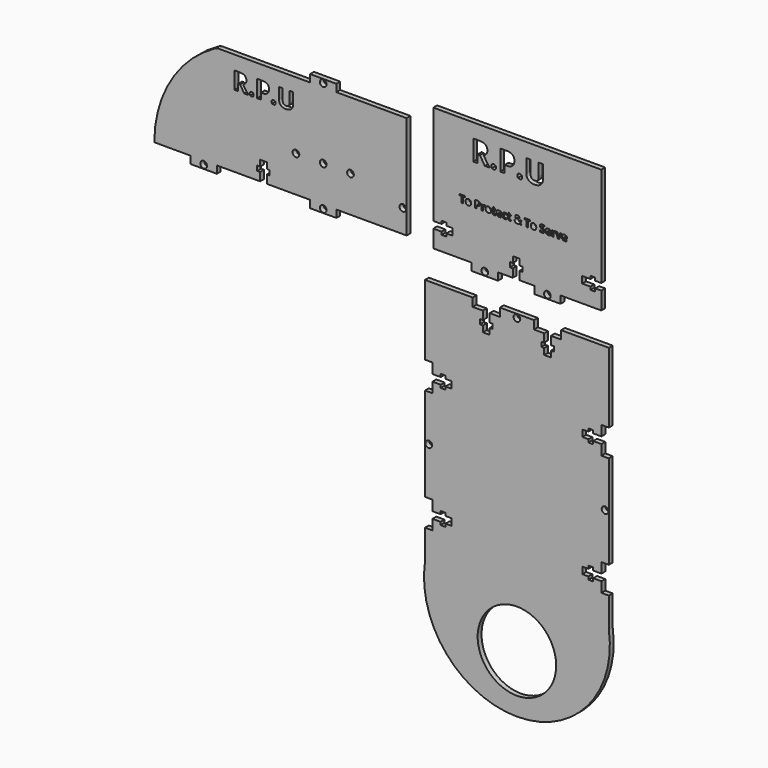
from build123d import *

# Parameters (mm, degrees)
F0_R     = 2.0574
F1_DEPTH = 2.9718
F2_R     = 2.0574
F3_DEPTH = 2.9718
F4_R     = 2.0574
F4_R_2   = 24.13
F5_DEPTH = 2.9718
F8_R     = 5.08


# Not quite as in the source:
# - ends of sketch curves that miss each other by under 0.0002 mm in the source are joined
# - a feature names something its author has since deleted; it is built from what else it names


with BuildPart() as f1:
    # F0 (on Front) → F1 (new body)
    with BuildSketch(Plane.XZ):
        Polygon((-18.5969026979, -10.7412008894), (-18.5969026979, -15.2876914638), (-2.4300471224, -15.2876914638), (-2.4300471224, -10.7412008894), (6.6548, -10.7412008894), (6.6548, -5.6612008894), (4.8768, -5.6612008894), (4.8768, -2.7392187621), (6.6548, -2.7392187621), (6.6548, 0.9935991106), (10.7696, 0.9935991106), (10.7696, -2.7392187621), (12.5476, -2.7392187621), (12.5476, -5.6612008894), (10.7696, -5.6612008894), (10.7696, -10.7412008894), (19.8544471224, -10.7412008894), (19.8544471224, -15.2876914638), (36.0213026979, -15.2876914638), (36.0213026979, -10.7412008894), (58.0559210762, -10.7412008894), (61.0555037856, -10.7412008894), (61.0555037856, -6.2738), (61.0555037856, 0), (57.3217037856, 0), (57.3217037856, -1.778), (54.4007037856, -1.778), (54.4007037856, 0), (49.3207037856, 0), (49.3207037856, 4.1148), (54.4007037856, 4.1148), (54.4007037856, 5.8928), (57.3051609099, 5.8928), (57.3051609099, 4.1148), (61.0555037856, 4.1148), (61.0555037856, 10.3886), (61.0555037856, 65.4587991106), (-42.2221365774, 65.4587991106), (-42.2221365774, 10.3886), (-42.2221365774, 4.1148), (-37.1421365774, 4.1148), (-37.1421365774, 5.8928905055), (-34.2144520407, 5.8928905055), (-34.2144520407, 4.1148), (-30.4746365774, 4.1148), (-30.4746365774, 0), (-34.2144520407, 0), (-34.2144520407, -1.7524508294), (-37.1421365774, -1.7524508294), (-37.1421365774, 0), (-42.2221365774, 0), (-42.2221365774, -6.2738), (-42.2221365774, -10.7412008894), (-38.2601322443, -10.7412008894), align=None)
        with Locations((-10.5134749102, -12.9762914638)):
            Circle(F0_R, mode=Mode.SUBTRACT)
        Polygon((-23.9621248782, 23.1793641805), (-23.9621248782, 19.4944459945), (-24.9110182404, 19.4944459945), (-24.9110182404, 23.1793641805), (-26.1262676342, 23.1793641805), (-26.1262676342, 23.9686397739), (-22.7478547345, 23.9686397739), (-22.7478547345, 23.1793641805), align=None, mode=Mode.SUBTRACT)
        with BuildLine():
            add(Edge.make_bspline(
                [(-19.2254920678, 22.1506619338), (-19.0237665439, 21.7496590113), (-19.0237665439, 21.2110714476)],
                knots=[0, 0, 0, 1, 1, 1], degree=2))
            add(Edge.make_bspline(
                [(-19.0237665439, 21.2110714476), (-19.0237665439, 20.3757710988), (-19.464429096, 19.904262168)],
                knots=[0, 0, 0, 1, 1, 1], degree=2))
            add(Edge.make_bspline(
                [(-19.464429096, 19.904262168), (-19.9050916482, 19.4327532372), (-20.6914294912, 19.4327532372)],
                knots=[0, 0, 0, 1, 1, 1], degree=2))
            add(Edge.make_bspline(
                [(-20.6914294912, 19.4327532372), (-21.1839922995, 19.4327532372), (-21.560513969, 19.6486778877)],
                knots=[0, 0, 0, 1, 1, 1], degree=2))
            add(Edge.make_bspline(
                [(-21.560513969, 19.6486778877), (-21.9370356386, 19.8646025383), (-22.1387611624, 20.2685432111)],
                knots=[0, 0, 0, 1, 1, 1], degree=2))
            add(Edge.make_bspline(
                [(-22.1387611624, 20.2685432111), (-22.3404866863, 20.6724838839), (-22.3404866863, 21.2110714476)],
                knots=[0, 0, 0, 1, 1, 1], degree=2))
            add(Edge.make_bspline(
                [(-22.3404866863, 21.2110714476), (-22.3404866863, 22.0493095468), (-21.9032515096, 22.5144533518)],
                knots=[0, 0, 0, 1, 1, 1], degree=2))
            add(Edge.make_bspline(
                [(-21.9032515096, 22.5144533518), (-21.4660163329, 22.9795971568), (-20.672823739, 22.9795971568)],
                knots=[0, 0, 0, 1, 1, 1], degree=2))
            add(Edge.make_bspline(
                [(-20.672823739, 22.9795971568), (-20.1802609307, 22.9795971568), (-19.8037392612, 22.7656310065)],
                knots=[0, 0, 0, 1, 1, 1], degree=2))
            add(Edge.make_bspline(
                [(-19.8037392612, 22.7656310065), (-19.4272175916, 22.5516648562), (-19.2254920678, 22.1506619338)],
                knots=[0, 0, 0, 1, 1, 1], degree=2))
        make_face(mode=Mode.SUBTRACT)
        with BuildLine():
            add(Edge.make_bspline(
                [(-13.8831930607, 23.6180682324), (-13.4596673856, 23.2674966909), (-13.4596673856, 22.5732083588)],
                knots=[0, 0, 0, 1, 1, 1], degree=2))
            add(Edge.make_bspline(
                [(-13.4596673856, 22.5732083588), (-13.4596673856, 21.8505217733), (-13.911101689, 21.468124603)],
                knots=[0, 0, 0, 1, 1, 1], degree=2))
            add(Edge.make_bspline(
                [(-13.911101689, 21.468124603), (-14.3625359924, 21.0857274328), (-15.1948985909, 21.0857274328)],
                knots=[0, 0, 0, 1, 1, 1], degree=2))
            Line((-15.1948985909, 21.0857274328), (-15.601287389, 21.0857274328))
            Line((-15.601287389, 21.0857274328), (-15.601287389, 19.4944459945))
            Line((-15.601287389, 19.4944459945), (-16.5501807512, 19.4944459945))
            Line((-16.5501807512, 19.4944459945), (-16.5501807512, 23.9686397739))
            Line((-16.5501807512, 23.9686397739), (-15.1214548322, 23.9686397739))
            add(Edge.make_bspline(
                [(-15.1214548322, 23.9686397739), (-14.3067187358, 23.9686397739), (-13.8831930607, 23.6180682324)],
                knots=[0, 0, 0, 1, 1, 1], degree=2))
        make_face(mode=Mode.SUBTRACT)
        with BuildLine():
            add(Edge.make_bspline(
                [(-11.367499513, 22.803821761), (-11.096736856, 22.9795971568), (-10.7784805684, 22.9795971568)],
                knots=[0, 0, 0, 1, 1, 1], degree=2))
            add(Edge.make_bspline(
                [(-10.7784805684, 22.9795971568), (-10.5885060459, 22.9795971568), (-10.4631620311, 22.9521781536)],
                knots=[0, 0, 0, 1, 1, 1], degree=2))
            Line((-10.4631620311, 22.9521781536), (-10.5336680394, 22.0777078001))
            add(Edge.make_bspline(
                [(-10.5336680394, 22.0777078001), (-10.6472610528, 22.1080645537), (-10.8088373219, 22.1080645537)],
                knots=[0, 0, 0, 1, 1, 1], degree=2))
            add(Edge.make_bspline(
                [(-10.8088373219, 22.1080645537), (-11.2553753748, 22.1080645537), (-11.5050841543, 21.8784304016)],
                knots=[0, 0, 0, 1, 1, 1], degree=2))
            add(Edge.make_bspline(
                [(-11.5050841543, 21.8784304016), (-11.7547929339, 21.6487962494), (-11.7547929339, 21.2355527005)],
                knots=[0, 0, 0, 1, 1, 1], degree=2))
            Line((-11.7547929339, 21.2355527005), (-11.7547929339, 19.4944459945))
            Line((-11.7547929339, 19.4944459945), (-12.6880182943, 19.4944459945))
            Line((-12.6880182943, 19.4944459945), (-12.6880182943, 22.9159458993))
            Line((-12.6880182943, 22.9159458993), (-11.9809997106, 22.9159458993))
            Line((-11.9809997106, 22.9159458993), (-11.8429254443, 22.3401468312))
            Line((-11.8429254443, 22.3401468312), (-11.797879939, 22.3401468312))
            add(Edge.make_bspline(
                [(-11.797879939, 22.3401468312), (-11.6382621701, 22.6280463652), (-11.367499513, 22.803821761)],
                knots=[0, 0, 0, 1, 1, 1], degree=2))
        make_face(mode=Mode.SUBTRACT)
        with BuildLine():
            add(Edge.make_bspline(
                [(-6.9349238636, 22.1506619338), (-6.7331983397, 21.7496590113), (-6.7331983397, 21.2110714476)],
                knots=[0, 0, 0, 1, 1, 1], degree=2))
            add(Edge.make_bspline(
                [(-6.7331983397, 21.2110714476), (-6.7331983397, 20.3757710988), (-7.1738608919, 19.904262168)],
                knots=[0, 0, 0, 1, 1, 1], degree=2))
            add(Edge.make_bspline(
                [(-7.1738608919, 19.904262168), (-7.614523444, 19.4327532372), (-8.400861287, 19.4327532372)],
                knots=[0, 0, 0, 1, 1, 1], degree=2))
            add(Edge.make_bspline(
                [(-8.400861287, 19.4327532372), (-8.8934240953, 19.4327532372), (-9.2699457649, 19.6486778877)],
                knots=[0, 0, 0, 1, 1, 1], degree=2))
            add(Edge.make_bspline(
                [(-9.2699457649, 19.6486778877), (-9.6464674344, 19.8646025383), (-9.8481929583, 20.2685432111)],
                knots=[0, 0, 0, 1, 1, 1], degree=2))
            add(Edge.make_bspline(
                [(-9.8481929583, 20.2685432111), (-10.0499184822, 20.6724838839), (-10.0499184822, 21.2110714476)],
                knots=[0, 0, 0, 1, 1, 1], degree=2))
            add(Edge.make_bspline(
                [(-10.0499184822, 21.2110714476), (-10.0499184822, 22.0493095468), (-9.6126833054, 22.5144533518)],
                knots=[0, 0, 0, 1, 1, 1], degree=2))
            add(Edge.make_bspline(
                [(-9.6126833054, 22.5144533518), (-9.1754481287, 22.9795971568), (-8.3822555348, 22.9795971568)],
                knots=[0, 0, 0, 1, 1, 1], degree=2))
            add(Edge.make_bspline(
                [(-8.3822555348, 22.9795971568), (-7.8896927266, 22.9795971568), (-7.513171057, 22.7656310065)],
                knots=[0, 0, 0, 1, 1, 1], degree=2))
            add(Edge.make_bspline(
                [(-7.513171057, 22.7656310065), (-7.1366493875, 22.5516648562), (-6.9349238636, 22.1506619338)],
                knots=[0, 0, 0, 1, 1, 1], degree=2))
        make_face(mode=Mode.SUBTRACT)
        with BuildLine():
            add(Edge.make_bspline(
                [(-4.8158266129, 20.2719705865), (-4.7041920997, 20.1769833253), (-4.5200930779, 20.1769833253)],
                knots=[0, 0, 0, 1, 1, 1], degree=2))
            add(Edge.make_bspline(
                [(-4.5200930779, 20.1769833253), (-4.2752805489, 20.1769833253), (-3.9325430084, 20.2837215879)],
                knots=[0, 0, 0, 1, 1, 1], degree=2))
            Line((-3.9325430084, 20.2837215879), (-3.9325430084, 19.5894332557))
            add(Edge.make_bspline(
                [(-3.9325430084, 19.5894332557), (-4.2811560496, 19.4327532372), (-4.7893868598, 19.4327532372)],
                knots=[0, 0, 0, 1, 1, 1], degree=2))
            add(Edge.make_bspline(
                [(-4.7893868598, 19.4327532372), (-5.349517926, 19.4327532372), (-5.6051022063, 19.7162461457)],
                knots=[0, 0, 0, 1, 1, 1], degree=2))
            add(Edge.make_bspline(
                [(-5.6051022063, 19.7162461457), (-5.8606864865, 19.9997390543), (-5.8606864865, 20.5657456212)],
                knots=[0, 0, 0, 1, 1, 1], degree=2))
            Line((-5.8606864865, 20.5657456212), (-5.8606864865, 22.2148028164))
            Line((-5.8606864865, 22.2148028164), (-6.3072245393, 22.2148028164))
            Line((-6.3072245393, 22.2148028164), (-6.3072245393, 22.609440613))
            Line((-6.3072245393, 22.609440613), (-5.7931182285, 22.9218214))
            Line((-5.7931182285, 22.9218214), (-5.5238244467, 23.6445079855))
            Line((-5.5238244467, 23.6445079855), (-4.9274611261, 23.6445079855))
            Line((-4.9274611261, 23.6445079855), (-4.9274611261, 22.9159458993))
            Line((-4.9274611261, 22.9159458993), (-3.9697545128, 22.9159458993))
            Line((-3.9697545128, 22.9159458993), (-3.9697545128, 22.2148028164))
            Line((-3.9697545128, 22.2148028164), (-4.9274611261, 22.2148028164))
            Line((-4.9274611261, 22.2148028164), (-4.9274611261, 20.5657456212))
            add(Edge.make_bspline(
                [(-4.9274611261, 20.5657456212), (-4.9274611261, 20.3669578477), (-4.8158266129, 20.2719705865)],
                knots=[0, 0, 0, 1, 1, 1], degree=2))
        make_face(mode=Mode.SUBTRACT)
        with BuildLine():
            add(Edge.make_bspline(
                [(-1.013398413, 19.4924874943), (-1.2915054459, 19.4327532372), (-1.6929979934, 19.4327532372)],
                knots=[0, 0, 0, 1, 1, 1], degree=2))
            add(Edge.make_bspline(
                [(-1.6929979934, 19.4327532372), (-2.5185058411, 19.4327532372), (-2.9836496461, 19.8890837912)],
                knots=[0, 0, 0, 1, 1, 1], degree=2))
            add(Edge.make_bspline(
                [(-2.9836496461, 19.8890837912), (-3.4487934511, 20.3454143452), (-3.4487934511, 21.180714694)],
                knots=[0, 0, 0, 1, 1, 1], degree=2))
            add(Edge.make_bspline(
                [(-3.4487934511, 21.180714694), (-3.4487934511, 22.0404962957), (-3.0189026503, 22.5100467263)],
                knots=[0, 0, 0, 1, 1, 1], degree=2))
            add(Edge.make_bspline(
                [(-3.0189026503, 22.5100467263), (-2.5890118494, 22.9795971568), (-1.8300930096, 22.9795971568)],
                knots=[0, 0, 0, 1, 1, 1], degree=2))
            add(Edge.make_bspline(
                [(-1.8300930096, 22.9795971568), (-1.1054479239, 22.9795971568), (-0.7015072511, 22.566843233)],
                knots=[0, 0, 0, 1, 1, 1], degree=2))
            add(Edge.make_bspline(
                [(-0.7015072511, 22.566843233), (-0.2975665783, 22.1540893092), (-0.2975665783, 21.425527223)],
                knots=[0, 0, 0, 1, 1, 1], degree=2))
            Line((-0.2975665783, 21.425527223), (-0.2975665783, 20.9721344193))
            Line((-0.2975665783, 20.9721344193), (-2.5038170893, 20.9721344193))
            add(Edge.make_bspline(
                [(-2.5038170893, 20.9721344193), (-2.4881490875, 20.5745588723), (-2.2678178114, 20.3512898459)],
                knots=[0, 0, 0, 1, 1, 1], degree=2))
            add(Edge.make_bspline(
                [(-2.2678178114, 20.3512898459), (-2.0474865354, 20.1280208195), (-1.6499109883, 20.1280208195)],
                knots=[0, 0, 0, 1, 1, 1], degree=2))
            add(Edge.make_bspline(
                [(-1.6499109883, 20.1280208195), (-1.3404679517, 20.1280208195), (-1.0652986691, 20.192161702)],
                knots=[0, 0, 0, 1, 1, 1], degree=2))
            add(Edge.make_bspline(
                [(-1.0652986691, 20.192161702), (-0.7901293866, 20.2563025846), (-0.4904788511, 20.3973146013)],
                knots=[0, 0, 0, 1, 1, 1], degree=2))
            Line((-0.4904788511, 20.3973146013), (-0.4904788511, 19.6746280158))
            add(Edge.make_bspline(
                [(-0.4904788511, 19.6746280158), (-0.7352913801, 19.5522217513), (-1.013398413, 19.4924874943)],
                knots=[0, 0, 0, 1, 1, 1], degree=2))
        make_face(mode=Mode.SUBTRACT)
        with BuildLine():
            add(Edge.make_bspline(
                [(2.4335619948, 19.4880808687), (2.2024589675, 19.4327532372), (1.8509081759, 19.4327532372)],
                knots=[0, 0, 0, 1, 1, 1], degree=2))
            add(Edge.make_bspline(
                [(1.8509081759, 19.4327532372), (0.2537512369, 19.4327532372), (0.2537512369, 21.1865901947)],
                knots=[0, 0, 0, 1, 1, 1], degree=2))
            add(Edge.make_bspline(
                [(0.2537512369, 21.1865901947), (0.2537512369, 22.0591020479), (0.6880486633, 22.5193496024)],
                knots=[0, 0, 0, 1, 1, 1], degree=2))
            add(Edge.make_bspline(
                [(0.6880486633, 22.5193496024), (1.1223460897, 22.9795971568), (1.9331651856, 22.9795971568)],
                knots=[0, 0, 0, 1, 1, 1], degree=2))
            add(Edge.make_bspline(
                [(1.9331651856, 22.9795971568), (2.5265907558, 22.9795971568), (2.9985893117, 22.7475148794)],
                knots=[0, 0, 0, 1, 1, 1], degree=2))
            Line((2.9985893117, 22.7475148794), (2.722440779, 22.0248282939))
            add(Edge.make_bspline(
                [(2.722440779, 22.0248282939), (2.5021095029, 22.1139400544), (2.3126246055, 22.1707365611)],
                knots=[0, 0, 0, 1, 1, 1], degree=2))
            add(Edge.make_bspline(
                [(2.3126246055, 22.1707365611), (2.1231397081, 22.2275330679), (1.9331651856, 22.2275330679)],
                knots=[0, 0, 0, 1, 1, 1], degree=2))
            add(Edge.make_bspline(
                [(1.9331651856, 22.2275330679), (1.2046030994, 22.2275330679), (1.2046030994, 21.1924656954)],
                knots=[0, 0, 0, 1, 1, 1], degree=2))
            add(Edge.make_bspline(
                [(1.2046030994, 21.1924656954), (1.2046030994, 20.1887343266), (1.9331651856, 20.1887343266)],
                knots=[0, 0, 0, 1, 1, 1], degree=2))
            add(Edge.make_bspline(
                [(1.9331651856, 20.1887343266), (2.2024589675, 20.1887343266), (2.4320931196, 20.2607092102)],
                knots=[0, 0, 0, 1, 1, 1], degree=2))
            add(Edge.make_bspline(
                [(2.4320931196, 20.2607092102), (2.6617272718, 20.3326840937), (2.8908717989, 20.4864263619)],
                knots=[0, 0, 0, 1, 1, 1], degree=2))
            Line((2.8908717989, 20.4864263619), (2.8908717989, 19.6873582673))
            add(Edge.make_bspline(
                [(2.8908717989, 19.6873582673), (2.6646650222, 19.5434085003), (2.4335619948, 19.4880808687)],
                knots=[0, 0, 0, 1, 1, 1], degree=2))
        make_face(mode=Mode.SUBTRACT)
        with BuildLine():
            add(Edge.make_bspline(
                [(4.8297870283, 20.2719705865), (4.9414215415, 20.1769833253), (5.1255205633, 20.1769833253)],
                knots=[0, 0, 0, 1, 1, 1], degree=2))
            add(Edge.make_bspline(
                [(5.1255205633, 20.1769833253), (5.3703330923, 20.1769833253), (5.7130706328, 20.2837215879)],
                knots=[0, 0, 0, 1, 1, 1], degree=2))
            Line((5.7130706328, 20.2837215879), (5.7130706328, 19.5894332557))
            add(Edge.make_bspline(
                [(5.7130706328, 19.5894332557), (5.3644575916, 19.4327532372), (4.8562267815, 19.4327532372)],
                knots=[0, 0, 0, 1, 1, 1], degree=2))
            add(Edge.make_bspline(
                [(4.8562267815, 19.4327532372), (4.2960957152, 19.4327532372), (4.0405114349, 19.7162461457)],
                knots=[0, 0, 0, 1, 1, 1], degree=2))
            add(Edge.make_bspline(
                [(4.0405114349, 19.7162461457), (3.7849271547, 19.9997390543), (3.7849271547, 20.5657456212)],
                knots=[0, 0, 0, 1, 1, 1], degree=2))
            Line((3.7849271547, 20.5657456212), (3.7849271547, 22.2148028164))
            Line((3.7849271547, 22.2148028164), (3.3383891019, 22.2148028164))
            Line((3.3383891019, 22.2148028164), (3.3383891019, 22.609440613))
            Line((3.3383891019, 22.609440613), (3.8524954127, 22.9218214))
            Line((3.8524954127, 22.9218214), (4.1217891946, 23.6445079855))
            Line((4.1217891946, 23.6445079855), (4.7181525151, 23.6445079855))
            Line((4.7181525151, 23.6445079855), (4.7181525151, 22.9159458993))
            Line((4.7181525151, 22.9159458993), (5.6758591284, 22.9159458993))
            Line((5.6758591284, 22.9159458993), (5.6758591284, 22.2148028164))
            Line((5.6758591284, 22.2148028164), (4.7181525151, 22.2148028164))
            Line((4.7181525151, 22.2148028164), (4.7181525151, 20.5657456212))
            add(Edge.make_bspline(
                [(4.7181525151, 20.5657456212), (4.7181525151, 20.3669578477), (4.8297870283, 20.2719705865)],
                knots=[0, 0, 0, 1, 1, 1], degree=2))
        make_face(mode=Mode.SUBTRACT)
        with Locations((27.9378749102, -12.9762914638)):
            Circle(F0_R, mode=Mode.SUBTRACT)
        with BuildLine():
            Line((11.3222152965, 20.3914391006), (12.2436896555, 19.4944459945))
            Line((12.2436896555, 19.4944459945), (11.090133019, 19.4944459945))
            Line((11.090133019, 19.4944459945), (10.7385822274, 19.8401212854))
            add(Edge.make_bspline(
                [(10.7385822274, 19.8401212854), (10.1539699083, 19.4327532372), (9.416594571, 19.4327532372)],
                knots=[0, 0, 0, 1, 1, 1], degree=2))
            add(Edge.make_bspline(
                [(9.416594571, 19.4327532372), (8.6694267326, 19.4327532372), (8.2317019308, 19.7759804028)],
                knots=[0, 0, 0, 1, 1, 1], degree=2))
            add(Edge.make_bspline(
                [(8.2317019308, 19.7759804028), (7.793977129, 20.1192075684), (7.793977129, 20.7028406375)],
                knots=[0, 0, 0, 1, 1, 1], degree=2))
            add(Edge.make_bspline(
                [(7.793977129, 20.7028406375), (7.793977129, 21.1229389372), (7.9790554009, 21.4181828471)],
                knots=[0, 0, 0, 1, 1, 1], degree=2))
            add(Edge.make_bspline(
                [(7.9790554009, 21.4181828471), (8.1641336728, 21.713426757), (8.6145887261, 21.9699902874)],
                knots=[0, 0, 0, 1, 1, 1], degree=2))
            add(Edge.make_bspline(
                [(8.6145887261, 21.9699902874), (8.3844649489, 22.2334085686), (8.2806644366, 22.473814472)],
                knots=[0, 0, 0, 1, 1, 1], degree=2))
            add(Edge.make_bspline(
                [(8.2806644366, 22.473814472), (8.1768639243, 22.7142203754), (8.1768639243, 22.998202909)],
                knots=[0, 0, 0, 1, 1, 1], degree=2))
            add(Edge.make_bspline(
                [(8.1768639243, 22.998202909), (8.1768639243, 23.4633467141), (8.5333109665, 23.7478188727)],
                knots=[0, 0, 0, 1, 1, 1], degree=2))
            add(Edge.make_bspline(
                [(8.5333109665, 23.7478188727), (8.8897580087, 24.0322910314), (9.4861213292, 24.0322910314)],
                knots=[0, 0, 0, 1, 1, 1], degree=2))
            add(Edge.make_bspline(
                [(9.4861213292, 24.0322910314), (10.0560448967, 24.0322910314), (10.3973135621, 23.7678935001)],
                knots=[0, 0, 0, 1, 1, 1], degree=2))
            add(Edge.make_bspline(
                [(10.3973135621, 23.7678935001), (10.7385822274, 23.5034959688), (10.7385822274, 23.0598956663)],
                knots=[0, 0, 0, 1, 1, 1], degree=2))
            add(Edge.make_bspline(
                [(10.7385822274, 23.0598956663), (10.7385822274, 22.6956146232), (10.5270642024, 22.3940055876)],
                knots=[0, 0, 0, 1, 1, 1], degree=2))
            add(Edge.make_bspline(
                [(10.5270642024, 22.3940055876), (10.3155461774, 22.0923965519), (9.8445268717, 21.8201650197)],
                knots=[0, 0, 0, 1, 1, 1], degree=2))
            Line((9.8445268717, 21.8201650197), (10.7141009745, 20.9721344193))
            add(Edge.make_bspline(
                [(10.7141009745, 20.9721344193), (10.9305152501, 21.3305399617), (11.090133019, 21.8936087784)],
                knots=[0, 0, 0, 1, 1, 1], degree=2))
            Line((11.090133019, 21.8936087784), (12.0635076342, 21.8936087784))
            add(Edge.make_bspline(
                [(12.0635076342, 21.8936087784), (11.9528523711, 21.4803652295), (11.7599400983, 21.0871963079)],
                knots=[0, 0, 0, 1, 1, 1], degree=2))
            add(Edge.make_bspline(
                [(11.7599400983, 21.0871963079), (11.5670278254, 20.6940273864), (11.3222152965, 20.3914391006)],
                knots=[0, 0, 0, 1, 1, 1], degree=2))
        make_face(mode=Mode.SUBTRACT)
        Polygon((16.1616693691, 23.1793641805), (16.1616693691, 19.4944459945), (15.2127760068, 19.4944459945), (15.2127760068, 23.1793641805), (13.997526613, 23.1793641805), (13.997526613, 23.9686397739), (17.3759395127, 23.9686397739), (17.3759395127, 23.1793641805), align=None, mode=Mode.SUBTRACT)
        with BuildLine():
            add(Edge.make_bspline(
                [(20.8983021795, 22.1506619338), (21.1000277033, 21.7496590113), (21.1000277033, 21.2110714476)],
                knots=[0, 0, 0, 1, 1, 1], degree=2))
            add(Edge.make_bspline(
                [(21.1000277033, 21.2110714476), (21.1000277033, 20.3757710988), (20.6593651512, 19.904262168)],
                knots=[0, 0, 0, 1, 1, 1], degree=2))
            add(Edge.make_bspline(
                [(20.6593651512, 19.904262168), (20.2187025991, 19.4327532372), (19.432364756, 19.4327532372)],
                knots=[0, 0, 0, 1, 1, 1], degree=2))
            add(Edge.make_bspline(
                [(19.432364756, 19.4327532372), (18.9398019478, 19.4327532372), (18.5632802782, 19.6486778877)],
                knots=[0, 0, 0, 1, 1, 1], degree=2))
            add(Edge.make_bspline(
                [(18.5632802782, 19.6486778877), (18.1867586087, 19.8646025383), (17.9850330848, 20.2685432111)],
                knots=[0, 0, 0, 1, 1, 1], degree=2))
            add(Edge.make_bspline(
                [(17.9850330848, 20.2685432111), (17.7833075609, 20.6724838839), (17.7833075609, 21.2110714476)],
                knots=[0, 0, 0, 1, 1, 1], degree=2))
            add(Edge.make_bspline(
                [(17.7833075609, 21.2110714476), (17.7833075609, 22.0493095468), (18.2205427377, 22.5144533518)],
                knots=[0, 0, 0, 1, 1, 1], degree=2))
            add(Edge.make_bspline(
                [(18.2205427377, 22.5144533518), (18.6577779144, 22.9795971568), (19.4509705082, 22.9795971568)],
                knots=[0, 0, 0, 1, 1, 1], degree=2))
            add(Edge.make_bspline(
                [(19.4509705082, 22.9795971568), (19.9435333165, 22.9795971568), (20.3200549861, 22.7656310065)],
                knots=[0, 0, 0, 1, 1, 1], degree=2))
            add(Edge.make_bspline(
                [(20.3200549861, 22.7656310065), (20.6965766556, 22.5516648562), (20.8983021795, 22.1506619338)],
                knots=[0, 0, 0, 1, 1, 1], degree=2))
        make_face(mode=Mode.SUBTRACT)
        with BuildLine():
            add(Edge.make_bspline(
                [(25.982079156, 21.4759586039), (26.2146510585, 21.1748391933), (26.2146510585, 20.7371143915)],
                knots=[0, 0, 0, 1, 1, 1], degree=2))
            add(Edge.make_bspline(
                [(26.2146510585, 20.7371143915), (26.2146510585, 20.1309585698), (25.7783951319, 19.7818559035)],
                knots=[0, 0, 0, 1, 1, 1], degree=2))
            add(Edge.make_bspline(
                [(25.7783951319, 19.7818559035), (25.3421392052, 19.4327532372), (24.5655938634, 19.4327532372)],
                knots=[0, 0, 0, 1, 1, 1], degree=2))
            add(Edge.make_bspline(
                [(24.5655938634, 19.4327532372), (23.8487827786, 19.4327532372), (23.2984442134, 19.7030262692)],
                knots=[0, 0, 0, 1, 1, 1], degree=2))
            Line((23.2984442134, 19.7030262692), (23.2984442134, 20.5843513734))
            add(Edge.make_bspline(
                [(23.2984442134, 20.5843513734), (23.750857767, 20.3816465995), (24.0647074291, 20.2993895897)],
                knots=[0, 0, 0, 1, 1, 1], degree=2))
            add(Edge.make_bspline(
                [(24.0647074291, 20.2993895897), (24.3785570912, 20.21713258), (24.6390376221, 20.21713258)],
                knots=[0, 0, 0, 1, 1, 1], degree=2))
            add(Edge.make_bspline(
                [(24.6390376221, 20.21713258), (24.9504391589, 20.21713258), (25.1174013037, 20.3361114691)],
                knots=[0, 0, 0, 1, 1, 1], degree=2))
            add(Edge.make_bspline(
                [(25.1174013037, 20.3361114691), (25.2843634484, 20.4550903582), (25.2843634484, 20.6910896361)],
                knots=[0, 0, 0, 1, 1, 1], degree=2))
            add(Edge.make_bspline(
                [(25.2843634484, 20.6910896361), (25.2843634484, 20.8223091516), (25.2109196897, 20.9251304138)],
                knots=[0, 0, 0, 1, 1, 1], degree=2))
            add(Edge.make_bspline(
                [(25.2109196897, 20.9251304138), (25.137475931, 21.0279516759), (24.9949950392, 21.1224493121)],
                knots=[0, 0, 0, 1, 1, 1], degree=2))
            add(Edge.make_bspline(
                [(24.9949950392, 21.1224493121), (24.8525141473, 21.2169469483), (24.4147893455, 21.425527223)],
                knots=[0, 0, 0, 1, 1, 1], degree=2))
            add(Edge.make_bspline(
                [(24.4147893455, 21.425527223), (24.0054627971, 21.6184394958), (23.8003098978, 21.7956837668)],
                knots=[0, 0, 0, 1, 1, 1], degree=2))
            add(Edge.make_bspline(
                [(23.8003098978, 21.7956837668), (23.5951569986, 21.9729280377), (23.4727507341, 22.2089273157)],
                knots=[0, 0, 0, 1, 1, 1], degree=2))
            add(Edge.make_bspline(
                [(23.4727507341, 22.2089273157), (23.3503444696, 22.4449265936), (23.3503444696, 22.7592658808)],
                knots=[0, 0, 0, 1, 1, 1], degree=2))
            add(Edge.make_bspline(
                [(23.3503444696, 22.7592658808), (23.3503444696, 23.3536707011), (23.7528162672, 23.6929808662)],
                knots=[0, 0, 0, 1, 1, 1], degree=2))
            add(Edge.make_bspline(
                [(23.7528162672, 23.6929808662), (24.1552880648, 24.0322910314), (24.8652443988, 24.0322910314)],
                knots=[0, 0, 0, 1, 1, 1], degree=2))
            add(Edge.make_bspline(
                [(24.8652443988, 24.0322910314), (25.2138574401, 24.0322910314), (25.5306448526, 23.9500340217)],
                knots=[0, 0, 0, 1, 1, 1], degree=2))
            add(Edge.make_bspline(
                [(25.5306448526, 23.9500340217), (25.847432265, 23.8677770119), (26.1931075559, 23.7179517442)],
                knots=[0, 0, 0, 1, 1, 1], degree=2))
            Line((26.1931075559, 23.7179517442), (25.8875815198, 22.9795971568))
            add(Edge.make_bspline(
                [(25.8875815198, 22.9795971568), (25.5291759774, 23.1264846742), (25.2951351997, 23.1847500561)],
                knots=[0, 0, 0, 1, 1, 1], degree=2))
            add(Edge.make_bspline(
                [(25.2951351997, 23.1847500561), (25.061094422, 23.243015438), (24.8348876452, 23.243015438)],
                knots=[0, 0, 0, 1, 1, 1], degree=2))
            add(Edge.make_bspline(
                [(24.8348876452, 23.243015438), (24.5655938634, 23.243015438), (24.4216440963, 23.1176714232)],
                knots=[0, 0, 0, 1, 1, 1], degree=2))
            add(Edge.make_bspline(
                [(24.4216440963, 23.1176714232), (24.2776943293, 22.9923274083), (24.2776943293, 22.7906018845)],
                knots=[0, 0, 0, 1, 1, 1], degree=2))
            add(Edge.make_bspline(
                [(24.2776943293, 22.7906018845), (24.2776943293, 22.6652578697), (24.3359597112, 22.5717394836)],
                knots=[0, 0, 0, 1, 1, 1], degree=2))
            add(Edge.make_bspline(
                [(24.3359597112, 22.5717394836), (24.3942250931, 22.4782210975), (24.5210379831, 22.3910678372)],
                knots=[0, 0, 0, 1, 1, 1], degree=2))
            add(Edge.make_bspline(
                [(24.5210379831, 22.3910678372), (24.6478508731, 22.3039145769), (25.1218079292, 22.0777078001)],
                knots=[0, 0, 0, 1, 1, 1], degree=2))
            add(Edge.make_bspline(
                [(25.1218079292, 22.0777078001), (25.7495072534, 21.7770780146), (25.982079156, 21.4759586039)],
                knots=[0, 0, 0, 1, 1, 1], degree=2))
        make_face(mode=Mode.SUBTRACT)
        with BuildLine():
            add(Edge.make_bspline(
                [(29.1798204093, 19.4924874943), (28.9017133764, 19.4327532372), (28.5002208289, 19.4327532372)],
                knots=[0, 0, 0, 1, 1, 1], degree=2))
            add(Edge.make_bspline(
                [(28.5002208289, 19.4327532372), (27.6747129812, 19.4327532372), (27.2095691762, 19.8890837912)],
                knots=[0, 0, 0, 1, 1, 1], degree=2))
            add(Edge.make_bspline(
                [(27.2095691762, 19.8890837912), (26.7444253712, 20.3454143452), (26.7444253712, 21.180714694)],
                knots=[0, 0, 0, 1, 1, 1], degree=2))
            add(Edge.make_bspline(
                [(26.7444253712, 21.180714694), (26.7444253712, 22.0404962957), (27.174316172, 22.5100467263)],
                knots=[0, 0, 0, 1, 1, 1], degree=2))
            add(Edge.make_bspline(
                [(27.174316172, 22.5100467263), (27.6042069729, 22.9795971568), (28.3631258127, 22.9795971568)],
                knots=[0, 0, 0, 1, 1, 1], degree=2))
            add(Edge.make_bspline(
                [(28.3631258127, 22.9795971568), (29.0877708984, 22.9795971568), (29.4917115712, 22.566843233)],
                knots=[0, 0, 0, 1, 1, 1], degree=2))
            add(Edge.make_bspline(
                [(29.4917115712, 22.566843233), (29.895652244, 22.1540893092), (29.895652244, 21.425527223)],
                knots=[0, 0, 0, 1, 1, 1], degree=2))
            Line((29.895652244, 21.425527223), (29.895652244, 20.9721344193))
            Line((29.895652244, 20.9721344193), (27.689401733, 20.9721344193))
            add(Edge.make_bspline(
                [(27.689401733, 20.9721344193), (27.7050697348, 20.5745588723), (27.9254010109, 20.3512898459)],
                knots=[0, 0, 0, 1, 1, 1], degree=2))
            add(Edge.make_bspline(
                [(27.9254010109, 20.3512898459), (28.145732287, 20.1280208195), (28.543307834, 20.1280208195)],
                knots=[0, 0, 0, 1, 1, 1], degree=2))
            add(Edge.make_bspline(
                [(28.543307834, 20.1280208195), (28.8527508706, 20.1280208195), (29.1279201532, 20.192161702)],
                knots=[0, 0, 0, 1, 1, 1], degree=2))
            add(Edge.make_bspline(
                [(29.1279201532, 20.192161702), (29.4030894357, 20.2563025846), (29.7027399712, 20.3973146013)],
                knots=[0, 0, 0, 1, 1, 1], degree=2))
            Line((29.7027399712, 20.3973146013), (29.7027399712, 19.6746280158))
            add(Edge.make_bspline(
                [(29.7027399712, 19.6746280158), (29.4579274422, 19.5522217513), (29.1798204093, 19.4924874943)],
                knots=[0, 0, 0, 1, 1, 1], degree=2))
        make_face(mode=Mode.SUBTRACT)
        with BuildLine():
            add(Edge.make_bspline(
                [(31.975089865, 22.803821761), (32.2458525221, 22.9795971568), (32.5641088097, 22.9795971568)],
                knots=[0, 0, 0, 1, 1, 1], degree=2))
            add(Edge.make_bspline(
                [(32.5641088097, 22.9795971568), (32.7540833322, 22.9795971568), (32.879427347, 22.9521781536)],
                knots=[0, 0, 0, 1, 1, 1], degree=2))
            Line((32.879427347, 22.9521781536), (32.8089213387, 22.0777078001))
            add(Edge.make_bspline(
                [(32.8089213387, 22.0777078001), (32.6953283252, 22.1080645537), (32.5337520561, 22.1080645537)],
                knots=[0, 0, 0, 1, 1, 1], degree=2))
            add(Edge.make_bspline(
                [(32.5337520561, 22.1080645537), (32.0872140033, 22.1080645537), (31.8375052237, 21.8784304016)],
                knots=[0, 0, 0, 1, 1, 1], degree=2))
            add(Edge.make_bspline(
                [(31.8375052237, 21.8784304016), (31.5877964442, 21.6487962494), (31.5877964442, 21.2355527005)],
                knots=[0, 0, 0, 1, 1, 1], degree=2))
            Line((31.5877964442, 21.2355527005), (31.5877964442, 19.4944459945))
            Line((31.5877964442, 19.4944459945), (30.6545710838, 19.4944459945))
            Line((30.6545710838, 19.4944459945), (30.6545710838, 22.9159458993))
            Line((30.6545710838, 22.9159458993), (31.3615896674, 22.9159458993))
            Line((31.3615896674, 22.9159458993), (31.4996639338, 22.3401468312))
            Line((31.4996639338, 22.3401468312), (31.5447094391, 22.3401468312))
            add(Edge.make_bspline(
                [(31.5447094391, 22.3401468312), (31.704327208, 22.6280463652), (31.975089865, 22.803821761)],
                knots=[0, 0, 0, 1, 1, 1], degree=2))
        make_face(mode=Mode.SUBTRACT)
        with BuildLine():
            Line((35.2717353801, 19.4944459945), (34.3140287668, 19.4944459945))
            Line((34.3140287668, 19.4944459945), (33.0106468625, 22.9159458993))
            Line((33.0106468625, 22.9159458993), (33.9869592281, 22.9159458993))
            Line((33.9869592281, 22.9159458993), (34.6479530563, 20.9662589186))
            add(Edge.make_bspline(
                [(34.6479530563, 20.9662589186), (34.7576290692, 20.5961023748), (34.7860273226, 20.2660950858)],
                knots=[0, 0, 0, 1, 1, 1], degree=2))
            Line((34.7860273226, 20.2660950858), (34.8036538247, 20.2660950858))
            add(Edge.make_bspline(
                [(34.8036538247, 20.2660950858), (34.8193218265, 20.5598701206), (34.941728091, 20.9662589186)],
                knots=[0, 0, 0, 1, 1, 1], degree=2))
            Line((34.941728091, 20.9662589186), (35.5997841689, 22.9159458993))
            Line((35.5997841689, 22.9159458993), (36.5760965344, 22.9159458993))
            Line((36.5760965344, 22.9159458993), (35.2717353801, 19.4944459945))
        make_face(mode=Mode.SUBTRACT)
        with BuildLine():
            add(Edge.make_bspline(
                [(39.2935156059, 19.4924874943), (39.015408573, 19.4327532372), (38.6139160255, 19.4327532372)],
                knots=[0, 0, 0, 1, 1, 1], degree=2))
            add(Edge.make_bspline(
                [(38.6139160255, 19.4327532372), (37.7884081778, 19.4327532372), (37.3232643728, 19.8890837912)],
                knots=[0, 0, 0, 1, 1, 1], degree=2))
            add(Edge.make_bspline(
                [(37.3232643728, 19.8890837912), (36.8581205678, 20.3454143452), (36.8581205678, 21.180714694)],
                knots=[0, 0, 0, 1, 1, 1], degree=2))
            add(Edge.make_bspline(
                [(36.8581205678, 21.180714694), (36.8581205678, 22.0404962957), (37.2880113686, 22.5100467263)],
                knots=[0, 0, 0, 1, 1, 1], degree=2))
            add(Edge.make_bspline(
                [(37.2880113686, 22.5100467263), (37.7179021695, 22.9795971568), (38.4768210093, 22.9795971568)],
                knots=[0, 0, 0, 1, 1, 1], degree=2))
            add(Edge.make_bspline(
                [(38.4768210093, 22.9795971568), (39.201466095, 22.9795971568), (39.6054067678, 22.566843233)],
                knots=[0, 0, 0, 1, 1, 1], degree=2))
            add(Edge.make_bspline(
                [(39.6054067678, 22.566843233), (40.0093474406, 22.1540893092), (40.0093474406, 21.425527223)],
                knots=[0, 0, 0, 1, 1, 1], degree=2))
            Line((40.0093474406, 21.425527223), (40.0093474406, 20.9721344193))
            Line((40.0093474406, 20.9721344193), (37.8030969296, 20.9721344193))
            add(Edge.make_bspline(
                [(37.8030969296, 20.9721344193), (37.8187649314, 20.5745588723), (38.0390962075, 20.3512898459)],
                knots=[0, 0, 0, 1, 1, 1], degree=2))
            add(Edge.make_bspline(
                [(38.0390962075, 20.3512898459), (38.2594274836, 20.1280208195), (38.6570030306, 20.1280208195)],
                knots=[0, 0, 0, 1, 1, 1], degree=2))
            add(Edge.make_bspline(
                [(38.6570030306, 20.1280208195), (38.9664460672, 20.1280208195), (39.2416153498, 20.192161702)],
                knots=[0, 0, 0, 1, 1, 1], degree=2))
            add(Edge.make_bspline(
                [(39.2416153498, 20.192161702), (39.5167846323, 20.2563025846), (39.8164351678, 20.3973146013)],
                knots=[0, 0, 0, 1, 1, 1], degree=2))
            Line((39.8164351678, 20.3973146013), (39.8164351678, 19.6746280158))
            add(Edge.make_bspline(
                [(39.8164351678, 19.6746280158), (39.5716226388, 19.5522217513), (39.2935156059, 19.4924874943)],
                knots=[0, 0, 0, 1, 1, 1], degree=2))
        make_face(mode=Mode.SUBTRACT)
        with BuildLine():
            add(Edge.make_bspline(
                [(-6.1983052656, 44.3673295813), (-6.5922546055, 44.7489251092), (-6.5922546055, 45.4434838757)],
                knots=[0, 0, 0, 1, 1, 1], degree=2))
            add(Edge.make_bspline(
                [(-6.5922546055, 45.4434838757), (-6.5922546055, 46.1627502664), (-6.2065411403, 46.5319919822)],
                knots=[0, 0, 0, 1, 1, 1], degree=2))
            add(Edge.make_bspline(
                [(-6.2065411403, 46.5319919822), (-5.8208276751, 46.901233698), (-5.0823442434, 46.901233698)],
                knots=[0, 0, 0, 1, 1, 1], degree=2))
            add(Edge.make_bspline(
                [(-5.0823442434, 46.901233698), (-4.3713137275, 46.901233698), (-3.9814823249, 46.5237561075)],
                knots=[0, 0, 0, 1, 1, 1], degree=2))
            add(Edge.make_bspline(
                [(-3.9814823249, 46.5237561075), (-3.5916509223, 46.146278517), (-3.5916509223, 45.4434838757)],
                knots=[0, 0, 0, 1, 1, 1], degree=2))
            add(Edge.make_bspline(
                [(-3.5916509223, 45.4434838757), (-3.5916509223, 44.7653968586), (-3.9856002622, 44.375565456)],
                knots=[0, 0, 0, 1, 1, 1], degree=2))
            add(Edge.make_bspline(
                [(-3.9856002622, 44.375565456), (-4.3795496022, 43.9857340534), (-5.0823442434, 43.9857340534)],
                knots=[0, 0, 0, 1, 1, 1], degree=2))
            add(Edge.make_bspline(
                [(-5.0823442434, 43.9857340534), (-5.8043559256, 43.9857340534), (-6.1983052656, 44.3673295813)],
                knots=[0, 0, 0, 1, 1, 1], degree=2))
        make_face(mode=Mode.SUBTRACT)
        with BuildLine():
            Line((-13.5433328542, 49.0288346627), (-14.9571580114, 49.0288346627))
            Line((-14.9571580114, 49.0288346627), (-14.9571580114, 44.2163385451))
            Line((-14.9571580114, 44.2163385451), (-17.6173455402, 44.2163385451))
            Line((-17.6173455402, 44.2163385451), (-17.6173455402, 56.7595757166))
            Line((-17.6173455402, 56.7595757166), (-13.963362464, 56.7595757166))
            add(Edge.make_bspline(
                [(-13.963362464, 56.7595757166), (-11.4047507232, 56.7595757166), (-10.1789780383, 55.8289218752)],
                knots=[0, 0, 0, 1, 1, 1], degree=2))
            add(Edge.make_bspline(
                [(-10.1789780383, 55.8289218752), (-8.9532053535, 54.8982680339), (-8.9532053535, 53.0012715608)],
                knots=[0, 0, 0, 1, 1, 1], degree=2))
            add(Edge.make_bspline(
                [(-8.9532053535, 53.0012715608), (-8.9532053535, 51.8949190591), (-9.5612874356, 51.032897507)],
                knots=[0, 0, 0, 1, 1, 1], degree=2))
            add(Edge.make_bspline(
                [(-9.5612874356, 51.032897507), (-10.1693695178, 50.1708759548), (-11.2867031858, 49.6822140558)],
                knots=[0, 0, 0, 1, 1, 1], degree=2))
            add(Edge.make_bspline(
                [(-11.2867031858, 49.6822140558), (-8.4535622882, 45.4517197504), (-7.5970313192, 44.2163385451)],
                knots=[0, 0, 0, 1, 1, 1], degree=2))
            Line((-7.5970313192, 44.2163385451), (-10.5482197541, 44.2163385451))
            Line((-10.5482197541, 44.2163385451), (-13.5433328542, 49.0288346627))
        make_face(mode=Mode.SUBTRACT)
        with BuildLine():
            add(Edge.make_bspline(
                [(6.4684700264, 55.7767613354), (7.6558086294, 54.7939469543), (7.6558086294, 52.847535233)],
                knots=[0, 0, 0, 1, 1, 1], degree=2))
            add(Edge.make_bspline(
                [(7.6558086294, 52.847535233), (7.6558086294, 50.8215100563), (6.3902292168, 49.7494736992)],
                knots=[0, 0, 0, 1, 1, 1], degree=2))
            add(Edge.make_bspline(
                [(6.3902292168, 49.7494736992), (5.1246498042, 48.6774373421), (2.7911519719, 48.6774373421)],
                knots=[0, 0, 0, 1, 1, 1], degree=2))
            Line((2.7911519719, 48.6774373421), (1.6518559714, 48.6774373421))
            Line((1.6518559714, 48.6774373421), (1.6518559714, 44.2163385451))
            Line((1.6518559714, 44.2163385451), (-1.0083315574, 44.2163385451))
            Line((-1.0083315574, 44.2163385451), (-1.0083315574, 56.7595757166))
            Line((-1.0083315574, 56.7595757166), (2.9970488395, 56.7595757166))
            add(Edge.make_bspline(
                [(2.9970488395, 56.7595757166), (5.2811314235, 56.7595757166), (6.4684700264, 55.7767613354)],
                knots=[0, 0, 0, 1, 1, 1], degree=2))
        make_face(mode=Mode.SUBTRACT)
        with BuildLine():
            add(Edge.make_bspline(
                [(9.8451786544, 44.3673295813), (9.4512293144, 44.7489251092), (9.4512293144, 45.4434838757)],
                knots=[0, 0, 0, 1, 1, 1], degree=2))
            add(Edge.make_bspline(
                [(9.4512293144, 45.4434838757), (9.4512293144, 46.1627502664), (9.8369427797, 46.5319919822)],
                knots=[0, 0, 0, 1, 1, 1], degree=2))
            add(Edge.make_bspline(
                [(9.8369427797, 46.5319919822), (10.2226562449, 46.901233698), (10.9611396765, 46.901233698)],
                knots=[0, 0, 0, 1, 1, 1], degree=2))
            add(Edge.make_bspline(
                [(10.9611396765, 46.901233698), (11.6721701925, 46.901233698), (12.062001595, 46.5237561075)],
                knots=[0, 0, 0, 1, 1, 1], degree=2))
            add(Edge.make_bspline(
                [(12.062001595, 46.5237561075), (12.4518329976, 46.146278517), (12.4518329976, 45.4434838757)],
                knots=[0, 0, 0, 1, 1, 1], degree=2))
            add(Edge.make_bspline(
                [(12.4518329976, 45.4434838757), (12.4518329976, 44.7653968586), (12.0578836577, 44.375565456)],
                knots=[0, 0, 0, 1, 1, 1], degree=2))
            add(Edge.make_bspline(
                [(12.0578836577, 44.375565456), (11.6639343178, 43.9857340534), (10.9611396765, 43.9857340534)],
                knots=[0, 0, 0, 1, 1, 1], degree=2))
            add(Edge.make_bspline(
                [(10.9611396765, 43.9857340534), (10.2391279943, 43.9857340534), (9.8451786544, 44.3673295813)],
                knots=[0, 0, 0, 1, 1, 1], degree=2))
        make_face(mode=Mode.SUBTRACT)
        with BuildLine():
            Line((22.5929400476, 56.7595757166), (25.2448917017, 56.7595757166))
            Line((25.2448917017, 56.7595757166), (25.2448917017, 48.6444938433))
            add(Edge.make_bspline(
                [(25.2448917017, 48.6444938433), (25.2448917017, 47.2526310186), (24.6230831617, 46.2066749315)],
                knots=[0, 0, 0, 1, 1, 1], degree=2))
            add(Edge.make_bspline(
                [(24.6230831617, 46.2066749315), (24.0012746217, 45.1607188443), (22.8249171851, 44.6020520103)],
                knots=[0, 0, 0, 1, 1, 1], degree=2))
            add(Edge.make_bspline(
                [(22.8249171851, 44.6020520103), (21.6485597484, 44.0433851763), (20.0453094731, 44.0433851763)],
                knots=[0, 0, 0, 1, 1, 1], degree=2))
            add(Edge.make_bspline(
                [(20.0453094731, 44.0433851763), (17.6267076022, 44.0433851763), (16.2883779631, 45.2842569648)],
                knots=[0, 0, 0, 1, 1, 1], degree=2))
            add(Edge.make_bspline(
                [(16.2883779631, 45.2842569648), (14.950048324, 46.5251287533), (14.950048324, 48.6774373421)],
                knots=[0, 0, 0, 1, 1, 1], degree=2))
            Line((14.950048324, 48.6774373421), (14.950048324, 56.7595757166))
            Line((14.950048324, 56.7595757166), (17.5992546865, 56.7595757166))
            Line((17.5992546865, 56.7595757166), (17.5992546865, 49.0809952025))
            add(Edge.make_bspline(
                [(17.5992546865, 49.0809952025), (17.5992546865, 47.6314812549), (18.1826291446, 46.9533942378)],
                knots=[0, 0, 0, 1, 1, 1], degree=2))
            add(Edge.make_bspline(
                [(18.1826291446, 46.9533942378), (18.7660036027, 46.2753072206), (20.1139417622, 46.2753072206)],
                knots=[0, 0, 0, 1, 1, 1], degree=2))
            add(Edge.make_bspline(
                [(20.1139417622, 46.2753072206), (21.4179552568, 46.2753072206), (22.0054476522, 46.9575121751)],
                knots=[0, 0, 0, 1, 1, 1], degree=2))
            add(Edge.make_bspline(
                [(22.0054476522, 46.9575121751), (22.5929400476, 47.6397171296), (22.5929400476, 49.0974669519)],
                knots=[0, 0, 0, 1, 1, 1], degree=2))
            Line((22.5929400476, 49.0974669519), (22.5929400476, 56.7595757166))
        make_face(mode=Mode.SUBTRACT)
    extrude(amount=F1_DEPTH)


with BuildPart() as f3:
    # F2 (on Front) → F3 (new body)
    with BuildSketch(Plane.XZ):
        with BuildLine():
            Line((-79.1750495537, -9.0780625232), (-35.9950495537, -9.0780625232))
            Line((-35.9950495537, -9.0780625232), (-35.9950495537, -2.9524219789))
            Line((-35.9950495537, -2.9524219789), (-35.9950495537, 13.2019780211))
            Line((-35.9950495537, 13.2019780211), (-35.9950495537, 54.4219374768))
            Line((-35.9950495537, 54.4219374768), (-79.1750495537, 54.4219374768))
            Line((-79.1750495537, 54.4219374768), (-79.1750495537, 58.9685374768))
            Line((-79.1750495537, 58.9685374768), (-95.3294495537, 58.9685374768))
            Line((-95.3294495537, 58.9685374768), (-95.3294495537, 54.4219374768))
            Line((-95.3294495537, 54.4219374768), (-152.6318495537, 54.4219374768))
            ThreePointArc((-152.6318495537, 54.4219374768), (-180.7064304088, 28.0336952904), (-191.0620495537, -9.0780625232))
            Line((-191.0620495537, -9.0780625232), (-168.7862495537, -9.0780625232))
            Line((-168.7862495537, -9.0780625232), (-168.7862495537, -13.6246625232))
            Line((-168.7862495537, -13.6246625232), (-152.6318495537, -13.6246625232))
            Line((-152.6318495537, -13.6246625232), (-152.6318495537, -9.0780625232))
            Line((-152.6318495537, -9.0780625232), (-132.3118495537, -9.0780625232))
            Line((-132.3118495537, -9.0780625232), (-126.0380495537, -9.0780625232))
            Line((-126.0380495537, -9.0780625232), (-126.0380495537, -3.9980625232))
            Line((-126.0380495537, -3.9980625232), (-127.8160495537, -3.9980625232))
            Line((-127.8160495537, -3.9980625232), (-127.8160495537, -1.0770625232))
            Line((-127.8160495537, -1.0770625232), (-126.0380495537, -1.0770625232))
            Line((-126.0380495537, -1.0770625232), (-126.0380495537, 2.6567374768))
            Line((-126.0380495537, 2.6567374768), (-121.9232495537, 2.6567374768))
            Line((-121.9232495537, 2.6567374768), (-121.9232495537, -1.0770625232))
            Line((-121.9232495537, -1.0770625232), (-120.147973299, -1.0770625232))
            Line((-120.147973299, -1.0770625232), (-120.147973299, -3.9980625232))
            Line((-120.147973299, -3.9980625232), (-121.9232495537, -3.9980625232))
            Line((-121.9232495537, -3.9980625232), (-121.9232495537, -9.0780625232))
            Line((-121.9232495537, -9.0780625232), (-115.6494495537, -9.0780625232))
            Line((-115.6494495537, -9.0780625232), (-95.3294495537, -9.0780625232))
            Line((-95.3294495537, -9.0780625232), (-95.3294495537, -13.6246625232))
            Line((-95.3294495537, -13.6246625232), (-79.1750495537, -13.6246625232))
            Line((-79.1750495537, -13.6246625232), (-79.1750495537, -9.0780625232))
        make_face()
        with Locations((-160.7090495537, -11.3132625232)):
            Circle(F2_R, mode=Mode.SUBTRACT)
        with Locations((-87.2522495537, -11.3132625232)):
            Circle(F2_R, mode=Mode.SUBTRACT)
        with Locations((-104.0162495537, 13.2019780211)):
            Circle(F2_R, mode=Mode.SUBTRACT)
        with Locations((-87.2522495537, 13.2019780211)):
            Circle(F2_R, mode=Mode.SUBTRACT)
        with Locations((-70.4882495537, 13.2019780211)):
            Circle(F2_R, mode=Mode.SUBTRACT)
        with Locations((-38.3064495537, 5.1247780211)):
            Circle(F2_R, mode=Mode.SUBTRACT)
        with BuildLine():
            Line((-138.3338374265, 39.3555876532), (-139.5205210235, 39.3555876532))
            Line((-139.5205210235, 39.3555876532), (-139.5205210235, 35.3162549436))
            Line((-139.5205210235, 35.3162549436), (-141.7533295777, 35.3162549436))
            Line((-141.7533295777, 35.3162549436), (-141.7533295777, 45.8443274765))
            Line((-141.7533295777, 45.8443274765), (-138.6863861456, 45.8443274765))
            add(Edge.make_bspline(
                [(-138.6863861456, 45.8443274765), (-136.5388344711, 45.8443274765), (-135.5099913138, 45.0631901185)],
                knots=[0, 0, 0, 1, 1, 1], degree=2))
            add(Edge.make_bspline(
                [(-135.5099913138, 45.0631901185), (-134.4811481564, 44.2820527605), (-134.4811481564, 42.6898229246)],
                knots=[0, 0, 0, 1, 1, 1], degree=2))
            add(Edge.make_bspline(
                [(-134.4811481564, 42.6898229246), (-134.4811481564, 41.761214207), (-134.9915373151, 41.0376828489)],
                knots=[0, 0, 0, 1, 1, 1], degree=2))
            add(Edge.make_bspline(
                [(-134.9915373151, 41.0376828489), (-135.5019264738, 40.3141514907), (-136.4397521514, 39.9039967718)],
                knots=[0, 0, 0, 1, 1, 1], degree=2))
            add(Edge.make_bspline(
                [(-136.4397521514, 39.9039967718), (-134.0617764775, 36.3531629409), (-133.3428535994, 35.3162549436)],
                knots=[0, 0, 0, 1, 1, 1], degree=2))
            Line((-133.3428535994, 35.3162549436), (-135.819911593, 35.3162549436))
            Line((-135.819911593, 35.3162549436), (-138.3338374265, 39.3555876532))
        make_face(mode=Mode.SUBTRACT)
        with BuildLine():
            add(Edge.make_bspline(
                [(-132.1688433224, 35.4429881433), (-132.4995017615, 35.7632775025), (-132.4995017615, 36.346250221)],
                knots=[0, 0, 0, 1, 1, 1], degree=2))
            add(Edge.make_bspline(
                [(-132.4995017615, 36.346250221), (-132.4995017615, 36.9499610994), (-132.1757560424, 37.2598813786)],
                knots=[0, 0, 0, 1, 1, 1], degree=2))
            add(Edge.make_bspline(
                [(-132.1757560424, 37.2598813786), (-131.8520103232, 37.5698016578), (-131.2321697648, 37.5698016578)],
                knots=[0, 0, 0, 1, 1, 1], degree=2))
            add(Edge.make_bspline(
                [(-131.2321697648, 37.5698016578), (-130.6353716063, 37.5698016578), (-130.3081695272, 37.2529686586)],
                knots=[0, 0, 0, 1, 1, 1], degree=2))
            add(Edge.make_bspline(
                [(-130.3081695272, 37.2529686586), (-129.980967448, 36.9361356594), (-129.980967448, 36.346250221)],
                knots=[0, 0, 0, 1, 1, 1], degree=2))
            add(Edge.make_bspline(
                [(-129.980967448, 36.346250221), (-129.980967448, 35.7771029424), (-130.3116258872, 35.4499008633)],
                knots=[0, 0, 0, 1, 1, 1], degree=2))
            add(Edge.make_bspline(
                [(-130.3116258872, 35.4499008633), (-130.6422843263, 35.1226987841), (-131.2321697648, 35.1226987841)],
                knots=[0, 0, 0, 1, 1, 1], degree=2))
            add(Edge.make_bspline(
                [(-131.2321697648, 35.1226987841), (-131.8381848832, 35.1226987841), (-132.1688433224, 35.4429881433)],
                knots=[0, 0, 0, 1, 1, 1], degree=2))
        make_face(mode=Mode.SUBTRACT)
        with BuildLine():
            add(Edge.make_bspline(
                [(-121.5370799897, 45.0194095586), (-120.5404961923, 44.1944916408), (-120.5404961923, 42.560785485)],
                knots=[0, 0, 0, 1, 1, 1], degree=2))
            add(Edge.make_bspline(
                [(-120.5404961923, 42.560785485), (-120.5404961923, 40.8602563693), (-121.6027508296, 39.9604506517)],
                knots=[0, 0, 0, 1, 1, 1], degree=2))
            add(Edge.make_bspline(
                [(-121.6027508296, 39.9604506517), (-122.6650054668, 39.060644934), (-124.6236094618, 39.060644934)],
                knots=[0, 0, 0, 1, 1, 1], degree=2))
            Line((-124.6236094618, 39.060644934), (-125.5798690593, 39.060644934))
            Line((-125.5798690593, 39.060644934), (-125.5798690593, 35.3162549436))
            Line((-125.5798690593, 35.3162549436), (-127.8126776136, 35.3162549436))
            Line((-127.8126776136, 35.3162549436), (-127.8126776136, 45.8443274765))
            Line((-127.8126776136, 45.8443274765), (-124.4507914622, 45.8443274765))
            add(Edge.make_bspline(
                [(-124.4507914622, 45.8443274765), (-122.5336637872, 45.8443274765), (-121.5370799897, 45.0194095586)],
                knots=[0, 0, 0, 1, 1, 1], degree=2))
        make_face(mode=Mode.SUBTRACT)
        with BuildLine():
            add(Edge.make_bspline(
                [(-118.702864797, 35.4429881433), (-119.0335232362, 35.7632775025), (-119.0335232362, 36.346250221)],
                knots=[0, 0, 0, 1, 1, 1], degree=2))
            add(Edge.make_bspline(
                [(-119.0335232362, 36.346250221), (-119.0335232362, 36.9499610994), (-118.709777517, 37.2598813786)],
                knots=[0, 0, 0, 1, 1, 1], degree=2))
            add(Edge.make_bspline(
                [(-118.709777517, 37.2598813786), (-118.3860317979, 37.5698016578), (-117.7661912394, 37.5698016578)],
                knots=[0, 0, 0, 1, 1, 1], degree=2))
            add(Edge.make_bspline(
                [(-117.7661912394, 37.5698016578), (-117.169393081, 37.5698016578), (-116.8421910018, 37.2529686586)],
                knots=[0, 0, 0, 1, 1, 1], degree=2))
            add(Edge.make_bspline(
                [(-116.8421910018, 37.2529686586), (-116.5149889227, 36.9361356594), (-116.5149889227, 36.346250221)],
                knots=[0, 0, 0, 1, 1, 1], degree=2))
            add(Edge.make_bspline(
                [(-116.5149889227, 36.346250221), (-116.5149889227, 35.7771029424), (-116.8456473618, 35.4499008633)],
                knots=[0, 0, 0, 1, 1, 1], degree=2))
            add(Edge.make_bspline(
                [(-116.8456473618, 35.4499008633), (-117.176305801, 35.1226987841), (-117.7661912394, 35.1226987841)],
                knots=[0, 0, 0, 1, 1, 1], degree=2))
            add(Edge.make_bspline(
                [(-117.7661912394, 35.1226987841), (-118.3722063579, 35.1226987841), (-118.702864797, 35.4429881433)],
                knots=[0, 0, 0, 1, 1, 1], degree=2))
        make_face(mode=Mode.SUBTRACT)
        with BuildLine():
            Line((-108.0031263846, 45.8443274765), (-105.7772305503, 45.8443274765))
            Line((-105.7772305503, 45.8443274765), (-105.7772305503, 39.032994054))
            add(Edge.make_bspline(
                [(-105.7772305503, 39.032994054), (-105.7772305503, 37.8647443771), (-106.299140909, 36.9868289393)],
                knots=[0, 0, 0, 1, 1, 1], degree=2))
            add(Edge.make_bspline(
                [(-106.299140909, 36.9868289393), (-106.8210512676, 36.1089135016), (-107.8084181051, 35.6400006628)],
                knots=[0, 0, 0, 1, 1, 1], degree=2))
            add(Edge.make_bspline(
                [(-107.8084181051, 35.6400006628), (-108.7957849425, 35.171087824), (-110.1414610991, 35.171087824)],
                knots=[0, 0, 0, 1, 1, 1], degree=2))
            add(Edge.make_bspline(
                [(-110.1414610991, 35.171087824), (-112.1714965338, 35.171087824), (-113.294813531, 36.2126043013)],
                knots=[0, 0, 0, 1, 1, 1], degree=2))
            add(Edge.make_bspline(
                [(-113.294813531, 36.2126043013), (-114.4181305281, 37.2541207786), (-114.4181305281, 39.060644934)],
                knots=[0, 0, 0, 1, 1, 1], degree=2))
            Line((-114.4181305281, 39.060644934), (-114.4181305281, 45.8443274765))
            Line((-114.4181305281, 45.8443274765), (-112.1945389338, 45.8443274765))
            Line((-112.1945389338, 45.8443274765), (-112.1945389338, 39.3993682131))
            add(Edge.make_bspline(
                [(-112.1945389338, 39.3993682131), (-112.1945389338, 38.1827294962), (-111.704887935, 37.6135822177)],
                knots=[0, 0, 0, 1, 1, 1], degree=2))
            add(Edge.make_bspline(
                [(-111.704887935, 37.6135822177), (-111.2152369363, 37.0444349392), (-110.0838550992, 37.0444349392)],
                knots=[0, 0, 0, 1, 1, 1], degree=2))
            add(Edge.make_bspline(
                [(-110.0838550992, 37.0444349392), (-108.989341102, 37.0444349392), (-108.4962337433, 37.6170385777)],
                knots=[0, 0, 0, 1, 1, 1], degree=2))
            add(Edge.make_bspline(
                [(-108.4962337433, 37.6170385777), (-108.0031263846, 38.1896422162), (-108.0031263846, 39.4131936531)],
                knots=[0, 0, 0, 1, 1, 1], degree=2))
            Line((-108.0031263846, 39.4131936531), (-108.0031263846, 45.8443274765))
        make_face(mode=Mode.SUBTRACT)
        with Locations((-87.2522495537, 56.6571374768)):
            Circle(F2_R, mode=Mode.SUBTRACT)
    extrude(amount=F3_DEPTH)


with BuildPart() as f5:
    # F4 (on Front) → F5 (new body)
    with BuildSketch(Plane.XZ):
        Polygon((-17.9715745272, -38.5677560119), (-47.3085745272, -38.5677560119), (-47.3085745272, -81.7477560119), (-42.7365745272, -81.7477560119), (-42.7365745272, -88.0215560119), (-37.6600883901, -88.0215560119), (-37.6600883901, -86.2435560119), (-34.7390883901, -86.2435560119), (-34.7529165447, -88.0215560119), (-31.0017745272, -88.0215560119), (-31.0017745272, -92.1363560119), (-34.7390883901, -92.1363560119), (-34.7390883901, -93.9143560119), (-37.6600883901, -93.9143560119), (-37.6600883901, -92.1363560119), (-42.7364388524, -92.1363560119), (-42.7364388524, -98.4101560119), (-47.3085745272, -98.4101560119), (-47.3085745272, -119.1156101778), (-47.3085745272, -135.2700101778), (-47.3085745272, -155.9710101778), (-42.7365745272, -155.9710101778), (-42.7365745272, -162.2448101778), (-37.6600883901, -162.2448101778), (-37.6600883901, -160.4668101778), (-34.7390883901, -160.4668101778), (-34.7390883901, -162.2448101778), (-31.0017745272, -162.2448101778), (-31.0017745272, -166.3596101778), (-34.7390883901, -166.3596101778), (-34.7390883901, -168.1283563375), (-37.6600883901, -168.1283563375), (-37.6600883901, -166.3596101778), (-42.7365745272, -166.3596101778), (-42.7365745272, -172.6334101778), (-47.3085745272, -172.6334101778), (-47.3085745272, -190.9677560119), (65.6960254728, -190.9677560119), (65.6960254728, -172.6334101778), (61.1240254728, -172.6334101778), (61.1240254728, -166.3596101778), (56.0475393357, -166.3596101778), (56.0475393357, -168.1283563375), (53.1265393357, -168.1283563375), (53.1265393357, -166.3596101778), (49.3892254728, -166.3596101778), (49.3892254728, -162.2448101778), (53.1265393357, -162.2448101778), (53.1265393357, -160.4668101778), (56.0475393357, -160.4668101778), (56.0475393357, -162.2448101778), (61.1240254728, -162.2448101778), (61.1240254728, -155.9710101778), (65.6960254728, -155.9710101778), (65.6960254728, -135.2700101778), (65.6960254728, -119.1156101778), (65.6960254728, -98.4101560119), (61.123889798, -98.4101560119), (61.123889798, -92.1363560119), (56.0475393357, -92.1363560119), (56.0475393357, -93.9143560119), (53.1265393357, -93.9143560119), (53.1265393357, -92.1363560119), (49.3892254728, -92.1363560119), (49.3892254728, -88.0215560119), (53.1403674903, -88.0215560119), (53.1265393357, -86.2435560119), (56.0475393357, -86.2435560119), (56.0475393357, -88.0215560119), (61.1240254728, -88.0215560119), (61.1240254728, -81.7477560119), (65.6960254728, -81.7477560119), (65.6960254728, -38.5677560119), (36.3590254728, -38.5677560119), (36.3590254728, -43.6396975759), (30.0852254728, -43.6396975759), (30.0852254728, -48.7235748508), (31.8632254728, -48.7235748508), (31.8632254728, -51.6445748508), (30.0852254728, -51.6445748508), (30.0852254728, -55.3871975759), (25.9704254728, -55.3871975759), (25.9704254728, -51.6445748508), (24.1924254728, -51.6445748508), (24.1924254728, -48.7235748508), (25.9704254728, -48.7235748508), (25.9704254728, -43.6435748508), (19.6966254728, -43.6435748508), (19.6966254728, -38.5677560119), (7.5744754728, -38.5677560119), (-1.3091745272, -38.5677560119), (-1.3091745272, -43.6435748508), (-7.5829745272, -43.6435748508), (-7.5829745272, -48.7235748508), (-5.8049745272, -48.7235748508), (-5.8049745272, -51.6445748508), (-7.5829745272, -51.6445748508), (-7.5829745272, -55.3871975759), (-11.6977745272, -55.3871975759), (-11.6977745272, -51.6445748508), (-13.4757745272, -51.6445748508), (-13.4757745272, -48.7235748508), (-11.6977745272, -48.7235748508), (-11.6977745272, -43.6396975759), (-17.9715745272, -43.6396975759), align=None)
        with Locations((-44.9971745272, -126.7686933279)):
            Circle(F4_R, mode=Mode.SUBTRACT)
        with BuildLine():
            ThreePointArc((11.2511254728, -40.8791560119), (8.243933193, -42.7042010484), (8.0132627478, -39.1941033377))
            ThreePointArc((8.0132627478, -39.1941033377), (10.1435177526, -39.0541109754), (11.2511254728, -40.8791560119))
        make_face(mode=Mode.SUBTRACT)
        with Locations((63.3846246285, -127.1948197924)):
            Circle(F4_R, mode=Mode.SUBTRACT)
        with BuildLine():
            Line((65.6960254728, -190.9677560119), (-47.3085745272, -190.9677560119))
            ThreePointArc((-47.3085745272, -190.9677560119), (9.1937254728, -256.5068706753), (65.6960254728, -190.9677560119))
        make_face()
        with Locations((9.1937254728, -221.0640013218)):
            Circle(F4_R_2, mode=Mode.SUBTRACT)
    extrude(amount=F5_DEPTH)


with BuildPart() as f3_1:
    # F6: moved
    add(f3.part.moved(Location((-22.606, 0, 0))))

    # F8
    f8_edges = [f3_1.edges().sort_by_distance(p)[0] for p in [
        (-175.23785, -1.4859, 54.421937),
    ]]
    fillet(f8_edges, radius=F8_R)


with BuildPart() as f5_1:
    # F7: moved
    add(f5.part.moved(Location((0, 0, 9.144))))


solid = Compound([f1.part, f3_1.part, f5_1.part])
